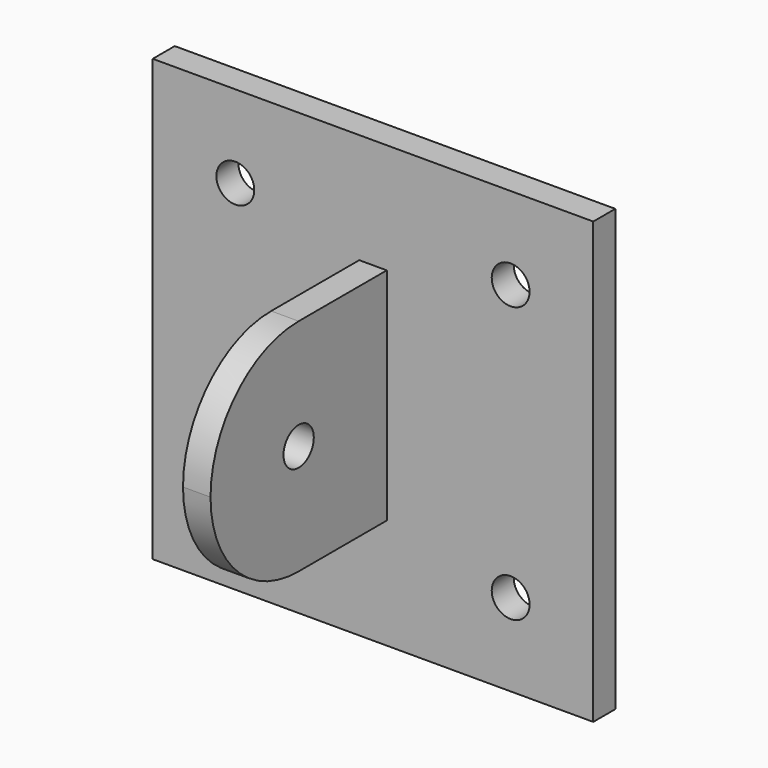
from build123d import *

# Parameters (mm, degrees)
F0_W            = 203.2
F0_H            = 203.2
F1_DEPTH        = 12.7
F2_W            = 12.7
F2_H            = 101.6
F3_DEPTH        = 101.6
F4_R            = 50.79999
F5_R            = 8.73125
F6_DEPTH        = 25.4
F7_R            = 8.73125
F8_DEPTH        = 25.4
F8_COPIES_COUNT = 4


# Not quite as in the source:
# - a fillet or chamfer is up to 0.001 mm smaller than in the source, because OpenCascade refuses the exact size
# - a pattern or mirror of a feature is missing from the dataset's text; its kind, count and spacing are read off the source's solid


with BuildPart() as f1:
    # F0 (on Front) → F1 (new body)
    with BuildSketch(Plane.XZ):
        Rectangle(F0_W, F0_H)
    extrude(amount=F1_DEPTH)

    # F2 (on face) → F3 (join)
    with BuildSketch(Plane.XZ.offset(12.7)):
        Rectangle(F2_W, F2_H)
    extrude(amount=F3_DEPTH)

    # F4 (radius 50.8 in the source; OpenCascade refuses exactly that, so slightly less here)
    f4_edges = [f1.edges().sort_by_distance(p)[0] for p in [
        (0, -114.3, 50.8),
        (0, -114.3, -50.8),
    ]]
    fillet(f4_edges, radius=F4_R)

    # F5 (on face) → F6 (cut)
    with BuildSketch(Plane.YZ.offset(6.35)):
        with Locations((-63.5, 0)):
            Circle(F5_R)
    extrude(amount=-F6_DEPTH, mode=Mode.SUBTRACT)

    # F7 (on face) → F8 (cut)
    with BuildSketch(Plane.XZ.offset(12.7)):
        with Locations((-63.5, 63.5)):
            Circle(F7_R)
    f8 = extrude(amount=-F8_DEPTH, mode=Mode.SUBTRACT)

    # F8_copies: F8 ×4 about axis
    f8_copies_axis = Axis((0, 0, 0), (0, 1, 0))
    for i in range(1, F8_COPIES_COUNT):
        add(f8.rotate(f8_copies_axis, i * 360 / F8_COPIES_COUNT), mode=Mode.SUBTRACT)


solid = f1.part
